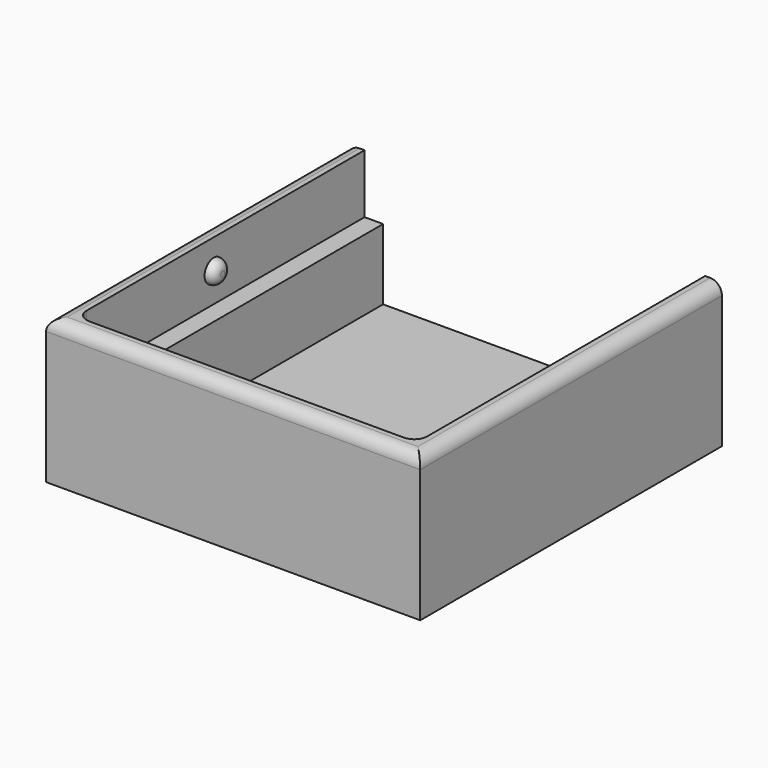
from build123d import *

# Parameters (mm, degrees)
F0_W      = 63.5
F0_H      = 64
F1_DEPTH  = 2.5
F3_DEPTH  = 12
F5_DEPTH  = 10
F6_R      = 2.2
F7_R      = 2
F8_R      = 1.95
F9_DEPTH  = 1.5
F10_R     = 1.49999
F11_R     = 1.95
F12_DEPTH = 1.5
F13_R     = 1.49999


# Not quite as in the source:
# - a fillet or chamfer is up to 0.001 mm smaller than in the source, because OpenCascade refuses the exact size


with BuildPart() as f1:
    # F0 (on Top) → F1 (new body)
    with BuildSketch(Plane.XY):
        Rectangle(F0_W, F0_H)
    extrude(amount=F1_DEPTH)

    # F2 (on face) → F3 (join)
    with BuildSketch(Plane.XY.offset(2.5)):
        Polygon((-25.75, 32), (-31.75, 32), (-31.75, -32), (31.75, -32), (31.75, 32), (25.75, 32), (25.75, -26), (-25.75, -26), align=None)
    extrude(amount=F3_DEPTH)

    # F4 (on face) → F5 (join)
    with BuildSketch(Plane.XY.offset(14.5)):
        Polygon((-28.9, 32), (-31.75, 32), (-31.75, -32), (31.75, -32), (31.75, 32), (28.9, 32), (28.9, -29.15), (-28.9, -29.15), align=None)
    extrude(amount=F5_DEPTH)

    # F6
    f6_edges = [f1.edges().sort_by_distance(p)[0] for p in [
        (-28.9, -29.15, 19.5),
        (28.9, -29.15, 19.5),
    ]]
    fillet(f6_edges, radius=F6_R)

    # F7
    f7_edges = [f1.edges().sort_by_distance(p)[0] for p in [
        (-31.75, 0, 24.5),
        (0, -32, 24.5),
        (31.75, 0, 24.5),
    ]]
    fillet(f7_edges, radius=F7_R)

    # F8 (on face) → F9 (join)
    with BuildSketch(Plane.YZ.offset(-28.9)):
        with Locations((0, 19.5)):
            Circle(F8_R)
    extrude(amount=F9_DEPTH)

    # F10 (radius 1.5 in the source; OpenCascade refuses exactly that, so slightly less here)
    f10_edges = [f1.edges().sort_by_distance(p)[0] for p in [
        (-27.4, -1.95, 19.5),
    ]]
    fillet(f10_edges, radius=F10_R)

    # F11 (on face) → F12 (join)
    with BuildSketch(Plane(origin=(28.9, 0, 0), x_dir=(0, -1, 0), z_dir=(-1, 0, 0))):
        with Locations((0, 19.5)):
            Circle(F11_R)
    extrude(amount=F12_DEPTH)

    # F13 (radius 1.5 in the source; OpenCascade refuses exactly that, so slightly less here)
    f13_edges = [f1.edges().sort_by_distance(p)[0] for p in [
        (27.4, 1.95, 19.5),
    ]]
    fillet(f13_edges, radius=F13_R)


solid = f1.part
